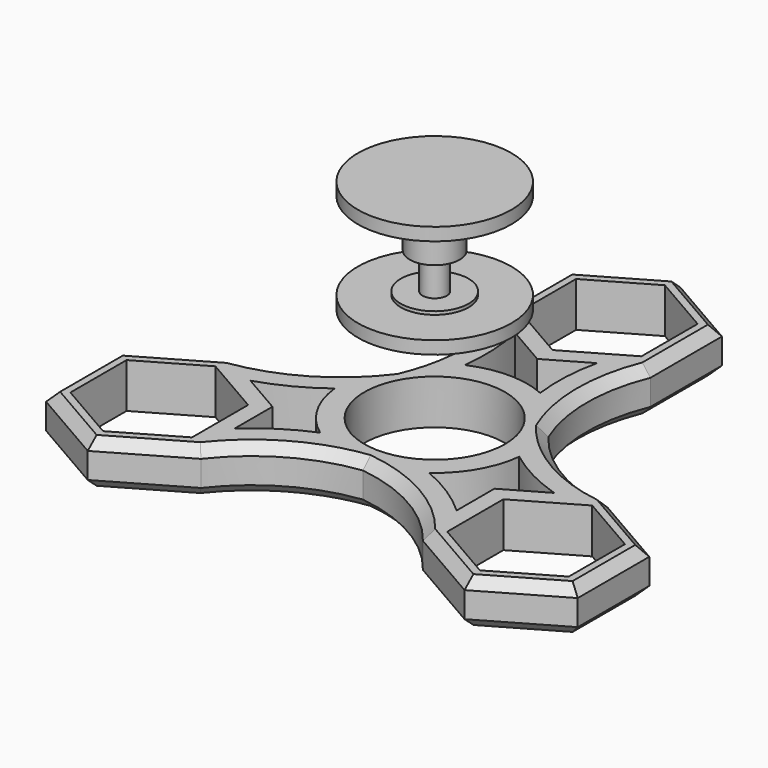
from build123d import *

# Parameters (mm, degrees)
F0_R        = 11
F1_DEPTH    = 7
F2_C1_SIZE  = 1.5
F2_C2_SIZE  = 1.5
F2_C3_SIZE  = 1.5
F2_C4_SIZE  = 1.5
F2_C5_SIZE  = 1.5
F2_C6_SIZE  = 1.5
F2_C7_SIZE  = 1.5
F2_C8_SIZE  = 1.5
F2_C9_SIZE  = 1.5
F2_C10_SIZE = 1.5
F2_C11_SIZE = 1.5
F2_C12_SIZE = 1.5
F2_C13_SIZE = 1.5
F2_C14_SIZE = 1.5
F2_C15_SIZE = 1.5
F2_C16_SIZE = 1.5
F2_C17_SIZE = 1.5
F2_C18_SIZE = 1.5
F2_C19_SIZE = 1.5
F2_C20_SIZE = 1.5
F2_C21_SIZE = 1.5
F2_C22_SIZE = 1.5
F2_C23_SIZE = 1.5
F2_C24_SIZE = 1.5
F2_C25_SIZE = 1.5
F2_C26_SIZE = 1.5
F2_C27_SIZE = 1.5
F2_C28_SIZE = 1.5
F2_C29_SIZE = 1.5
F2_C30_SIZE = 1.5
F2_C31_SIZE = 1.5
F2_C32_SIZE = 1.5
F2_C33_SIZE = 1.5
F2_C34_SIZE = 1.5
F2_C35_SIZE = 1.5
F2_C36_SIZE = 1.5


with BuildPart() as f1:
    # F0 (on Top) → F1 (new body)
    with BuildSketch(Plane.XY):
        with BuildLine():
            Line((-12.1000001989, 40.985938372), (-12.1000001989, 27.014061628))
            ThreePointArc((-12.1000001989, 27.014061628), (-10.1262410801, 17.0088965937), (-12.1471185409, 7.0131421595))
            ThreePointArc((-12.1471185409, 7.0131421595), (-19.7932570806, 0.2651337234), (-29.4448637287, -3.028123256))
            Line((-29.4448637287, -3.028123256), (-41.5448639275, -10.014061628))
            Line((-41.5448639275, -10.014061628), (-41.5448639275, -23.985938372))
            Line((-41.5448639275, -23.985938372), (-29.4448637287, -30.971876744))
            Line((-29.4448637287, -30.971876744), (-17.3448635298, -23.985938372))
            ThreePointArc((-17.3448635298, -23.985938372), (-9.6670160005, -17.2740303171), (0, -14.0262843189))
            ThreePointArc((0, -14.0262843189), (9.6670160005, -17.2740303171), (17.3448635298, -23.985938372))
            Line((17.3448635298, -23.985938372), (29.4448637287, -30.971876744))
            Line((29.4448637287, -30.971876744), (41.5448639275, -23.985938372))
            Line((41.5448639275, -23.985938372), (41.5448639275, -10.014061628))
            Line((41.5448639275, -10.014061628), (29.4448637287, -3.028123256))
            ThreePointArc((29.4448637287, -3.028123256), (19.7932570806, 0.2651337234), (12.1471185409, 7.0131421595))
            ThreePointArc((12.1471185409, 7.0131421595), (10.1262410801, 17.0088965937), (12.1000001989, 27.014061628))
            Line((12.1000001989, 27.014061628), (12.1000001989, 40.985938372))
            Line((12.1000001989, 40.985938372), (0, 47.971876744))
            Line((0, 47.971876744), (-12.1000001989, 40.985938372))
        make_face()
        Polygon((-29.4448637287, -27.9696551146), (-38.9448637287, -22.4848275573), (-38.9448637287, -11.5151724427), (-29.4448637287, -6.0303448854), (-19.9448637287, -11.5151724427), (-19.9448637287, -22.4848275573), align=None, mode=Mode.SUBTRACT)
        with BuildLine():
            Line((-17.3448635298, -17.39779537), (-17.3448635298, -10.014061628))
            Line((-17.3448635298, -10.014061628), (-23.7393645251, -6.322194757))
            ThreePointArc((-23.7393645251, -6.322194757), (-18.8718751166, -4.3202733927), (-14.4210197002, -1.5113539646))
            ThreePointArc((-14.4210197002, -1.5113539646), (-12.5573683549, -7.25), (-8.5193807775, -11.7332924266))
            ThreePointArc((-8.5193807775, -11.7332924266), (-13.1774040677, -14.1833865716), (-17.3448635298, -17.39779537))
        make_face(mode=Mode.SUBTRACT)
        Circle(F0_R, mode=Mode.SUBTRACT)
        Polygon((38.9448637287, -11.5151724427), (38.9448637287, -22.4848275573), (29.4448637287, -27.9696551146), (19.9448637287, -22.4848275573), (19.9448637287, -11.5151724427), (29.4448637287, -6.0303448854), align=None, mode=Mode.SUBTRACT)
        with BuildLine():
            Line((23.7393645251, -6.322194757), (17.3448635298, -10.014061628))
            Line((17.3448635298, -10.014061628), (17.3448635298, -17.39779537))
            ThreePointArc((17.3448635298, -17.39779537), (13.1774040677, -14.1833865716), (8.5193807775, -11.7332924266))
            ThreePointArc((8.5193807775, -11.7332924266), (12.5573683549, -7.25), (14.4210197002, -1.5113539646))
            ThreePointArc((14.4210197002, -1.5113539646), (18.8718751166, -4.3202733927), (23.7393645251, -6.322194757))
        make_face(mode=Mode.SUBTRACT)
        with BuildLine():
            ThreePointArc((6.3945009953, 23.719990127), (5.6944710489, 18.5036599644), (5.9016389227, 13.2446463911))
            ThreePointArc((5.9016389227, 13.2446463911), (0, 14.5), (-5.9016389227, 13.2446463911))
            ThreePointArc((-5.9016389227, 13.2446463911), (-5.6944710489, 18.5036599644), (-6.3945009953, 23.719990127))
            Line((-6.3945009953, 23.719990127), (0, 20.028123256))
            Line((0, 20.028123256), (6.3945009953, 23.719990127))
        make_face(mode=Mode.SUBTRACT)
        Polygon((9.5, 39.4848275573), (9.5, 28.5151724427), (0, 23.0303448854), (-9.5, 28.5151724427), (-9.5, 39.4848275573), (0, 44.9696551146), align=None, mode=Mode.SUBTRACT)
    extrude(amount=F1_DEPTH)

    # F2: chamfer of 1.5 on 36 edges, made by hand

    # F2_c1
    f2_c1_edges = [f1.edges().sort_by_distance(p)[0] for p in [
        (-12.1000001989, 34, 0),
    ]]
    chamfer(f2_c1_edges, length=F2_C1_SIZE)

    # F2_c2
    f2_c2_edges = [f1.edges().sort_by_distance(p)[0] for p in [
        (-12.1000001989, 34, 7),
    ]]
    chamfer(f2_c2_edges, length=F2_C2_SIZE)

    # F2_c3
    f2_c3_edges = [f1.edges().sort_by_distance(p)[0] for p in [
        (-10.2635253889, 14.3994277983, 0),
    ]]
    chamfer(f2_c3_edges, length=F2_C3_SIZE)

    # F2_c4
    f2_c4_edges = [f1.edges().sort_by_distance(p)[0] for p in [
        (-10.2635253889, 14.3994277983, 7),
    ]]
    chamfer(f2_c4_edges, length=F2_C4_SIZE)

    # F2_c5
    f2_c5_edges = [f1.edges().sort_by_distance(p)[0] for p in [
        (-19.7932570806, 0.2651337234, 0),
    ]]
    chamfer(f2_c5_edges, length=F2_C5_SIZE)

    # F2_c6
    f2_c6_edges = [f1.edges().sort_by_distance(p)[0] for p in [
        (-19.7932570806, 0.2651337234, 7),
    ]]
    chamfer(f2_c6_edges, length=F2_C6_SIZE)

    # F2_c7
    f2_c7_edges = [f1.edges().sort_by_distance(p)[0] for p in [
        (-36.9861521886, -7.3820881783, 0),
    ]]
    chamfer(f2_c7_edges, length=F2_C7_SIZE)

    # F2_c8
    f2_c8_edges = [f1.edges().sort_by_distance(p)[0] for p in [
        (-36.9861521886, -7.3820881783, 7),
    ]]
    chamfer(f2_c8_edges, length=F2_C8_SIZE)

    # F2_c9
    f2_c9_edges = [f1.edges().sort_by_distance(p)[0] for p in [
        (-41.5448639275, -17.8660254038, 0),
    ]]
    chamfer(f2_c9_edges, length=F2_C9_SIZE)

    # F2_c10
    f2_c10_edges = [f1.edges().sort_by_distance(p)[0] for p in [
        (-41.5448639275, -17.8660254038, 7),
    ]]
    chamfer(f2_c10_edges, length=F2_C10_SIZE)

    # F2_c11
    f2_c11_edges = [f1.edges().sort_by_distance(p)[0] for p in [
        (-34.7448638281, -27.9119202599, 0),
    ]]
    chamfer(f2_c11_edges, length=F2_C11_SIZE)

    # F2_c12
    f2_c12_edges = [f1.edges().sort_by_distance(p)[0] for p in [
        (-34.7448638281, -27.9119202599, 7),
    ]]
    chamfer(f2_c12_edges, length=F2_C12_SIZE)

    # F2_c13
    f2_c13_edges = [f1.edges().sort_by_distance(p)[0] for p in [
        (-22.6448636292, -27.0458948561, 0),
    ]]
    chamfer(f2_c13_edges, length=F2_C13_SIZE)

    # F2_c14
    f2_c14_edges = [f1.edges().sort_by_distance(p)[0] for p in [
        (-22.6448636292, -27.0458948561, 7),
    ]]
    chamfer(f2_c14_edges, length=F2_C14_SIZE)

    # F2_c15
    f2_c15_edges = [f1.edges().sort_by_distance(p)[0] for p in [
        (-7.3385075789, -16.0881876183, 0),
    ]]
    chamfer(f2_c15_edges, length=F2_C15_SIZE)

    # F2_c16
    f2_c16_edges = [f1.edges().sort_by_distance(p)[0] for p in [
        (-7.3385075789, -16.0881876183, 7),
    ]]
    chamfer(f2_c16_edges, length=F2_C16_SIZE)

    # F2_c17
    f2_c17_edges = [f1.edges().sort_by_distance(p)[0] for p in [
        (9.6670160005, -17.2740303171, 0),
    ]]
    chamfer(f2_c17_edges, length=F2_C17_SIZE)

    # F2_c18
    f2_c18_edges = [f1.edges().sort_by_distance(p)[0] for p in [
        (9.6670160005, -17.2740303171, 7),
    ]]
    chamfer(f2_c18_edges, length=F2_C18_SIZE)

    # F2_c19
    f2_c19_edges = [f1.edges().sort_by_distance(p)[0] for p in [
        (24.8861519897, -28.3399032944, 0),
    ]]
    chamfer(f2_c19_edges, length=F2_C19_SIZE)

    # F2_c20
    f2_c20_edges = [f1.edges().sort_by_distance(p)[0] for p in [
        (24.8861519897, -28.3399032944, 7),
    ]]
    chamfer(f2_c20_edges, length=F2_C20_SIZE)

    # F2_c21
    f2_c21_edges = [f1.edges().sort_by_distance(p)[0] for p in [
        (36.2448638281, -27.0458948561, 0),
    ]]
    chamfer(f2_c21_edges, length=F2_C21_SIZE)

    # F2_c22
    f2_c22_edges = [f1.edges().sort_by_distance(p)[0] for p in [
        (36.2448638281, -27.0458948561, 7),
    ]]
    chamfer(f2_c22_edges, length=F2_C22_SIZE)

    # F2_c23
    f2_c23_edges = [f1.edges().sort_by_distance(p)[0] for p in [
        (41.5448639275, -16.1339745962, 0),
    ]]
    chamfer(f2_c23_edges, length=F2_C23_SIZE)

    # F2_c24
    f2_c24_edges = [f1.edges().sort_by_distance(p)[0] for p in [
        (41.5448639275, -16.1339745962, 7),
    ]]
    chamfer(f2_c24_edges, length=F2_C24_SIZE)

    # F2_c25
    f2_c25_edges = [f1.edges().sort_by_distance(p)[0] for p in [
        (34.7448638281, -6.0880797401, 0),
    ]]
    chamfer(f2_c25_edges, length=F2_C25_SIZE)

    # F2_c26
    f2_c26_edges = [f1.edges().sort_by_distance(p)[0] for p in [
        (34.7448638281, -6.0880797401, 7),
    ]]
    chamfer(f2_c26_edges, length=F2_C26_SIZE)

    # F2_c27
    f2_c27_edges = [f1.edges().sort_by_distance(p)[0] for p in [
        (17.6020329678, 1.68875982, 0),
    ]]
    chamfer(f2_c27_edges, length=F2_C27_SIZE)

    # F2_c28
    f2_c28_edges = [f1.edges().sort_by_distance(p)[0] for p in [
        (17.6020329678, 1.68875982, 7),
    ]]
    chamfer(f2_c28_edges, length=F2_C28_SIZE)

    # F2_c29
    f2_c29_edges = [f1.edges().sort_by_distance(p)[0] for p in [
        (10.1262410801, 17.0088965937, 0),
    ]]
    chamfer(f2_c29_edges, length=F2_C29_SIZE)

    # F2_c30
    f2_c30_edges = [f1.edges().sort_by_distance(p)[0] for p in [
        (10.1262410801, 17.0088965937, 7),
    ]]
    chamfer(f2_c30_edges, length=F2_C30_SIZE)

    # F2_c31
    f2_c31_edges = [f1.edges().sort_by_distance(p)[0] for p in [
        (12.1000001989, 35.7219914727, 0),
    ]]
    chamfer(f2_c31_edges, length=F2_C31_SIZE)

    # F2_c32
    f2_c32_edges = [f1.edges().sort_by_distance(p)[0] for p in [
        (12.1000001989, 35.7219914727, 7),
    ]]
    chamfer(f2_c32_edges, length=F2_C32_SIZE)

    # F2_c33
    f2_c33_edges = [f1.edges().sort_by_distance(p)[0] for p in [
        (5.3000000994, 44.9119202599, 0),
    ]]
    chamfer(f2_c33_edges, length=F2_C33_SIZE)

    # F2_c34
    f2_c34_edges = [f1.edges().sort_by_distance(p)[0] for p in [
        (5.3000000994, 44.9119202599, 7),
    ]]
    chamfer(f2_c34_edges, length=F2_C34_SIZE)

    # F2_c35
    f2_c35_edges = [f1.edges().sort_by_distance(p)[0] for p in [
        (-6.0500000994, 44.478907558, 0),
    ]]
    chamfer(f2_c35_edges, length=F2_C35_SIZE)

    # F2_c36
    f2_c36_edges = [f1.edges().sort_by_distance(p)[0] for p in [
        (-6.0500000994, 44.478907558, 7),
    ]]
    chamfer(f2_c36_edges, length=F2_C36_SIZE)


with BuildPart() as f4:
    # F3 (on Front) → F4 (revolve)
    with BuildSketch(Plane.XZ):
        Polygon((12, 37.5604808674), (12, 39.5604808674), (0, 39.5604808674), (0, 38.3482346942), (0, 34.8104808674), (2, 34.8104808674), (2, 30.0604808674), (3.9, 30.0604808674), (3.9, 37.0604808674), (5.3, 37.0604808674), (5.3, 37.5604808674), align=None)
    revolve(axis=Axis((0, 0, 36.5793577808), (0, 0, 1)))

    # F3 (on Front) → F5 (revolve)
    with BuildSketch(Plane.XZ):
        Polygon((12, 37.5604808674), (12, 39.5604808674), (0, 39.5604808674), (0, 38.3482346942), (0, 34.8104808674), (2, 34.8104808674), (2, 30.0604808674), (3.9, 30.0604808674), (3.9, 37.0604808674), (5.3, 37.0604808674), (5.3, 37.5604808674), align=None)
    revolve(axis=Axis((0, 0, 30.0604808674), (0, 0, 1)))


with BuildPart() as f5:
    # F3 (on Front) → F5, piece 2 (revolve)
    with BuildSketch(Plane.XZ):
        Polygon((1.9, 29.1078351825), (0, 29.1078351825), (0, 21.9578351825), (12, 21.9578351825), (12, 23.9578351825), (5.3, 23.9578351825), (5.3, 24.4578351825), (1.9, 24.4578351825), align=None)
    revolve(axis=Axis((0, 0, 30.0604808674), (0, 0, 1)))


solid = Compound([f1.part, f4.part, f5.part])
